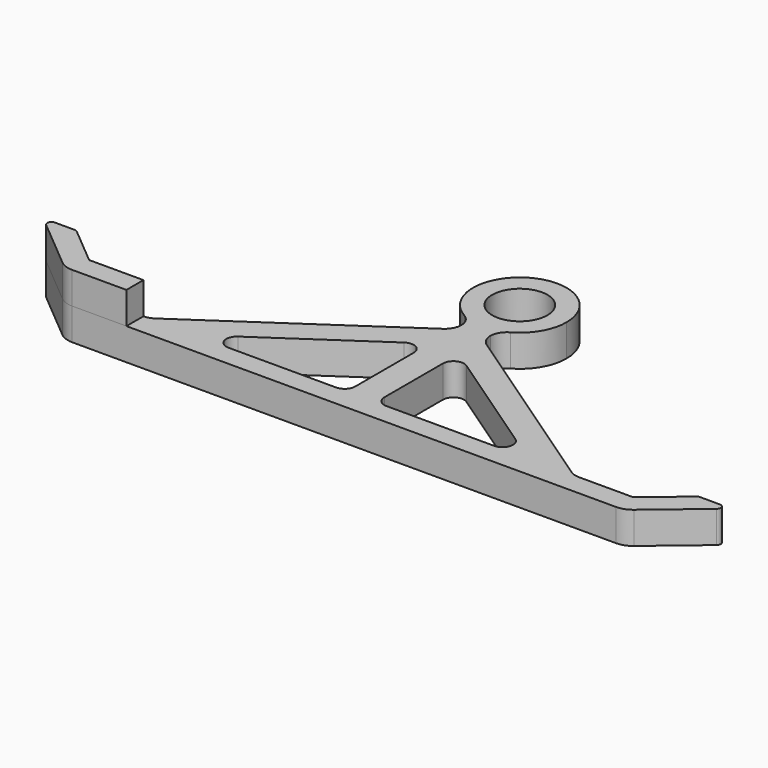
from build123d import *

# Parameters (mm, degrees)
F0_R        = 8.255
F1_DEPTH    = 9.525
F2_T1_DEPTH = 9.525
F4_DEPTH    = 9.525


# Not quite as in the source:
# - a fillet or chamfer that OpenCascade refuses, or shapes differently, is made with other operations: its cross-section is extruded or revolved along the edge and cut away or added
# - ends of sketch curves that miss each other by under 0.0002 mm in the source are joined
# - a feature names something its author has since deleted; it is built from what else it names


with BuildPart() as f1:
    # F0 (on Top) → F1 (new body)
    with BuildSketch(Plane.XY):
        with BuildLine():
            ThreePointArc((4.3122524784, 37.526747704), (-0.0112650872, 36.8307900709), (-4.3378264209, 37.5075678728))
            Line((-4.3378264209, 37.5075678728), (-4.3122524784, 31.736497147))
            Line((-4.3122524784, 31.736497147), (-63.5, -8.504387986))
            Line((-63.5, -8.504387986), (-81.28, -8.5043879861))
            Line((-81.28, -8.5043879861), (-92.6004192464, 0.9945716283))
            ThreePointArc((-92.6004192464, 0.9945716283), (-92.9823939286, 1.215104814), (-93.4167595107, 1.2916951856))
            Line((-93.4167595107, 1.2916951856), (-99.344067291, 1.2916951856))
            ThreePointArc((-99.344067291, 1.2916951856), (-100.5374769194, 0.4560607676), (-100.1604075553, -0.9511812572))
            Line((-100.1604075553, -0.9511812572), (-85.3617007511, -13.3687706785))
            ThreePointArc((-85.3617007511, -13.3687706785), (-83.4518273397, -14.4714366067), (-81.2799994295, -14.8543884647))
            Line((-81.2799994295, -14.8543884647), (55.6916793662, -14.8543884647))
            Line((55.6916793662, -14.8543884647), (81.2799994295, -14.8543884647))
            ThreePointArc((81.2799994295, -14.8543884647), (83.4518273397, -14.4714366067), (85.3617007511, -13.3687706785))
            Line((85.3617007511, -13.3687706785), (100.1604075553, -0.9511812572))
            ThreePointArc((100.1604075553, -0.9511812572), (100.5374769194, 0.4560607676), (99.344067291, 1.2916951856))
            Line((99.344067291, 1.2916951856), (93.4167595107, 1.2916951856))
            ThreePointArc((93.4167595107, 1.2916951856), (92.9823939286, 1.215104814), (92.6004192464, 0.9945716283))
            Line((92.6004192464, 0.9945716283), (81.2799994295, -8.5043884647))
            Line((81.2799994295, -8.5043884647), (63.5, -8.504387986))
            Line((63.5, -8.504387986), (4.3122524784, 31.736497147))
            Line((4.3122524784, 31.736497147), (4.3122524784, 37.526747704))
        make_face()
        with BuildLine():
            ThreePointArc((-9.272381027, 19.1498236636), (-6.0018498632, 19.3302933306), (-4.3122524784, 16.5241921081))
            Line((-4.3122524784, 16.5241921081), (-4.3122524784, -5.329387986))
            ThreePointArc((-4.3122524784, -5.329387986), (-5.2421884481, -7.5744520163), (-7.4872524784, -8.504387986))
            Line((-7.4872524784, -8.504387986), (-39.630287523, -8.504387986))
            ThreePointArc((-39.630287523, -8.504387986), (-42.6648389881, -6.2632629272), (-41.4154160715, -2.7037564306))
            Line((-41.4154160715, -2.7037564306), (-9.272381027, 19.1498236636))
        make_face(mode=Mode.SUBTRACT)
        with BuildLine():
            Line((4.3967338988, -5.3492686827), (4.3967338988, 16.5043114114))
            ThreePointArc((4.3967338988, 16.5043114114), (6.0757516386, 19.2928418474), (9.3258039242, 19.1135022159))
            Line((9.3258039242, 19.1135022159), (41.4688389688, -2.7400778782))
            ThreePointArc((41.4688389688, -2.7400778782), (42.7104384529, -6.2772960382), (39.6948882467, -8.504387986))
            Line((39.6948882467, -8.504387986), (7.5518532022, -8.504387986))
            ThreePointArc((7.5518532022, -8.504387986), (5.3208469473, -7.5802749375), (4.3967338988, -5.3492686827))
        make_face(mode=Mode.SUBTRACT)
        with BuildLine():
            ThreePointArc((4.3122524784, 37.526747704), (11.2713168612, 42.6053719635), (13.9277592898, 50.8007557298))
            ThreePointArc((13.9277592898, 50.8007557298), (-8.2626898349, 62.0961138999), (-4.3378264209, 37.5075678728))
            ThreePointArc((-4.3378264209, 37.5075678728), (-0.0112650872, 36.8307900709), (4.3122524784, 37.526747704))
        make_face()
        with Locations((-0.0422407102, 50.8007557298)):
            Circle(F0_R, mode=Mode.SUBTRACT)
    extrude(amount=F1_DEPTH)

    # F2: fillet of radius 5.08 on 6 edges, made by hand

    # F2_s2 → F2_t1 (join)
    with BuildSketch(Plane.XY):
        with BuildLine():
            ThreePointArc((6.5360468007, 30.2245718646), (4.9024905224, 32.0489381691), (4.3122524784, 34.4255823534))
            Line((4.3122524784, 34.4255823534), (4.3122524784, 31.736497147))
            Line((4.3122524784, 31.736497147), (6.5360468007, 30.2245718646))
        make_face()
        with BuildLine():
            ThreePointArc((4.3122524784, 34.2510476275), (4.9998161704, 36.8030866711), (6.8763876281, 38.6643031214))
            ThreePointArc((6.8763876281, 38.6643031214), (5.6229446638, 38.0310033956), (4.3122524784, 37.526747704))
            Line((4.3122524784, 37.526747704), (4.3122524784, 34.2510476275))
        make_face()
        with BuildLine():
            ThreePointArc((-4.3242327121, 34.4399823871), (-4.909166003, 32.0507806283), (-6.5479771563, 30.2164605901))
            Line((-6.5479771563, 30.2164605901), (-4.3122524784, 31.736497147))
            Line((-4.3122524784, 31.736497147), (-4.3242327121, 34.4399823871))
        make_face()
        with BuildLine():
            ThreePointArc((-6.9069886961, 38.6337456168), (-5.0221798353, 36.7808624145), (-4.3233105691, 34.2318896113))
            Line((-4.3233105691, 34.2318896113), (-4.3378264209, 37.5075678728))
            ThreePointArc((-4.3378264209, 37.5075678728), (-5.6507459596, 38.0060080235), (-6.9069886961, 38.6337456168))
        make_face()
        with BuildLine():
            ThreePointArc((65.063356077, -8.5043880281), (63.5691562425, -8.2796703522), (62.207150536, -7.6253985169))
            Line((62.207150536, -7.6253985169), (63.5, -8.504387986))
            Line((63.5, -8.504387986), (65.063356077, -8.5043880281))
        make_face()
        with BuildLine():
            ThreePointArc((-62.2071504741, -7.6253984748), (-63.569156246, -8.2796703302), (-65.0633561518, -8.504387986))
            Line((-65.0633561518, -8.504387986), (-63.5, -8.504387986))
            Line((-63.5, -8.504387986), (-62.2071504741, -7.6253984748))
        make_face()
    extrude(amount=F2_T1_DEPTH)


with BuildPart() as f4:
    # F3 (on face) → F4 (new body)
    with BuildSketch(Plane.XY.offset(9.525)):
        with BuildLine():
            ThreePointArc((-92.6004192464, 0.9945716283), (-92.9823939286, 1.215104814), (-93.4167595107, 1.2916951856))
            Line((-93.4167595107, 1.2916951856), (-99.344067291, 1.2916951856))
            ThreePointArc((-99.344067291, 1.2916951856), (-100.5374769194, 0.4560607676), (-100.1604075553, -0.9511812572))
            Line((-100.1604075553, -0.9511812572), (-85.3617007511, -13.3687706785))
            ThreePointArc((-85.3617007511, -13.3687706785), (-83.451827419, -14.4714365778), (-81.2799995983, -14.8543884647))
            Line((-81.2799995983, -14.8543884647), (-65.0633561518, -14.8543884647))
            Line((-65.0633561518, -14.8543884647), (-65.0633561518, -8.504387986))
            Line((-65.0633561518, -8.504387986), (-81.28, -8.5043879861))
            Line((-81.28, -8.5043879861), (-92.6004192464, 0.9945716283))
        make_face()
    extrude(amount=F4_DEPTH)


solid = Compound([f1.part, f4.part])
